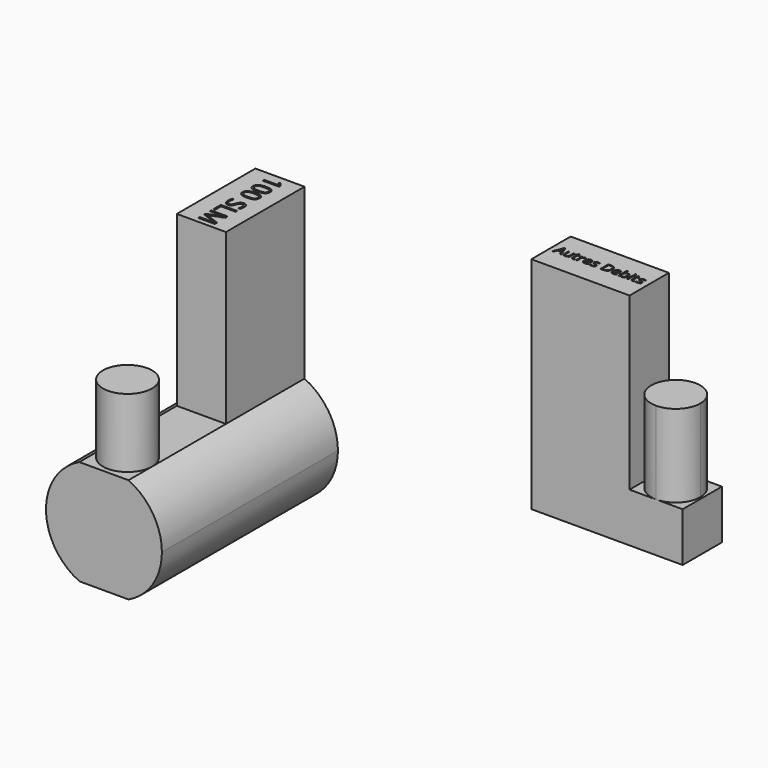
from build123d import *

# Parameters (mm, degrees)
F0_W          = 77
F0_H          = 25
F1_DEPTH      = 25
F2_W          = 50
F2_H          = 25
F3_DEPTH      = 87
F4_DEPTH      = 42
F5_TEXT_SIZE  = 7.1784817631
F6_DEPTH      = 2
F8_DEPTH      = 112
F9_W          = 25
F9_H          = 50
F10_DEPTH     = 86
F11_DEPTH     = 35
F12_TEXT_SIZE = 11.7259536988
F13_DEPTH     = 2


# Not quite as in the source:
# - Text() gives the source's letters only with a copy of the font that has no kerning and outlines rounded to 1/6400 em; it was checked with that copy


with BuildPart() as f1:
    # F0 (on Top) → F1 (new body)
    with BuildSketch(Plane.XY):
        with Locations((13.7132350355, 21.1470937739)):
            Rectangle(F0_W, F0_H)
    extrude(amount=F1_DEPTH)

    # F2 (on face) → F3 (join)
    with BuildSketch(Plane.XY.offset(25)):
        with Locations((0.2132350355, 21.1470937739)):
            Rectangle(F2_W, F2_H)
    extrude(amount=F3_DEPTH)

    # F2 (on face) → F4 (join)
    with BuildSketch(Plane.XY.offset(25)):
        with BuildLine():
            ThreePointArc((51.2132350355, 21.1470937739), (47.5520698004, 29.9859285387), (38.7132350355, 33.6470937739))
            ThreePointArc((38.7132350355, 33.6470937739), (26.2132350355, 21.1470937739), (38.7132350355, 8.6470937739))
            ThreePointArc((38.7132350355, 8.6470937739), (47.5520698004, 12.308259009), (51.2132350355, 21.1470937739))
        make_face()
    extrude(amount=F4_DEPTH)

    # F5 (on face) → F6 (cut)
    with BuildSketch(Plane.XY.offset(112)):
        with Locations((-22.5753320605, 19.1997186107)):
            Text('Autres Debits', F5_TEXT_SIZE, font='Open Sans', text_align=(TextAlign.LEFT, TextAlign.BOTTOM))
    extrude(amount=-F6_DEPTH, mode=Mode.SUBTRACT)


with BuildPart() as f8:
    # F7 (on Front) → F8 (new body)
    with BuildSketch(Plane.XZ):
        with BuildLine():
            ThreePointArc((-133.3279109196, -26.7207784318), (-120.9381539903, -15.8350876221), (-116.3279109196, 0))
            ThreePointArc((-116.3279109196, 0), (-120.9381539903, 15.8350876221), (-133.3279109196, 26.7207784318))
            Line((-133.3279109196, 26.7207784318), (-158.3279109196, 26.7207784318))
            ThreePointArc((-158.3279109196, 26.7207784318), (-175.3279109196, 0), (-158.3279109196, -26.7207784318))
            Line((-158.3279109196, -26.7207784318), (-133.3279109196, -26.7207784318))
        make_face()
    extrude(amount=F8_DEPTH)

    # F9 (on face) → F10 (join)
    with BuildSketch(Plane.XY.offset(26.7207784318)):
        with Locations((-145.8279109196, -25)):
            Rectangle(F9_W, F9_H)
    extrude(amount=F10_DEPTH)

    # F9 (on face) → F11 (join)
    with BuildSketch(Plane.XY.offset(26.7207784318)):
        with BuildLine():
            ThreePointArc((-158.3279109196, -97), (-145.8279109196, -109.5), (-133.3279109196, -97))
            ThreePointArc((-133.3279109196, -97), (-145.8279109196, -84.5), (-158.3279109196, -97))
        make_face()
    extrude(amount=F11_DEPTH)

    # F12 (on face) → F13 (cut)
    with BuildSketch(Plane.XY.offset(112.7207784318)):
        with Locations(Location((-149.5312877667, -2.2584988736), (0, 0, -90))):
            Text('100 SLM', F12_TEXT_SIZE, font='Open Sans', text_align=(TextAlign.LEFT, TextAlign.BOTTOM))
    extrude(amount=-F13_DEPTH, mode=Mode.SUBTRACT)


solid = Compound([f1.part, f8.part])
